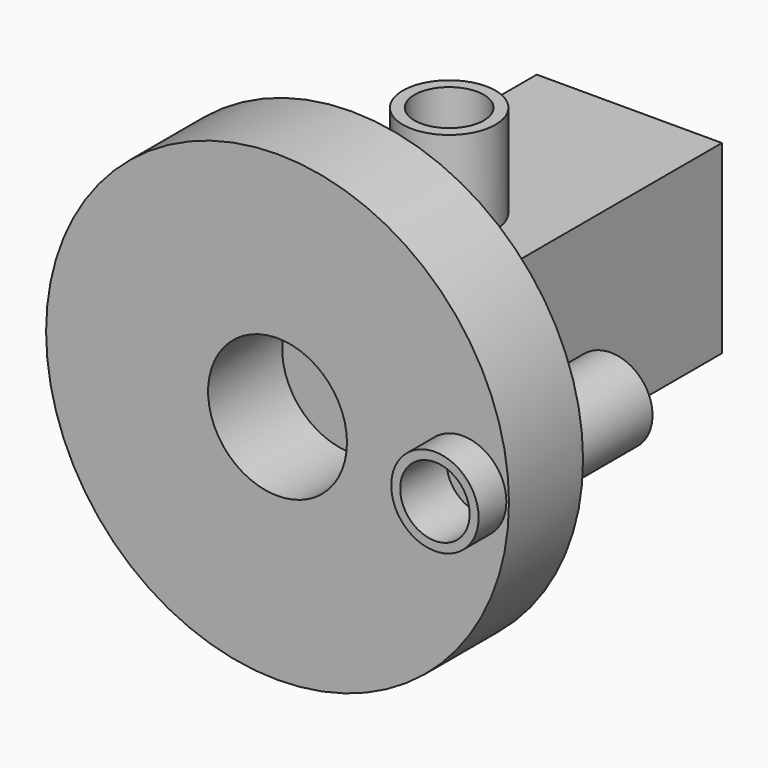
from build123d import *
from build123d import SkipClean  # not in build123d's __all__

# Parameters (mm, degrees)
F0_R      = 63.5
F1_DEPTH  = 25.4
F2_R      = 19.05
F3_DEPTH  = 25.401
F4_R      = 6.35
F5_DEPTH  = 25.4
F6_R      = 9.525
F7_DEPTH  = 6.35
F8_W      = 50.8
F8_H      = 50.8
F9_DEPTH  = 95.25
F10_R     = 19.05
F11_DEPTH = 88.9
F12_R     = 11.4435821265
F12_R_2   = 8.6754099319
F12_R_3   = 6.35
F13_DEPTH = 25.4
F14_R     = 12.7
F15_DEPTH = 25.4
F16_R     = 9.525
F17_DEPTH = 25.4
F18_R     = 11.9876896331
F18_R_2   = 9.525
F19_DEPTH = 9.525


# Not quite as in the source:
# - after a boolean that leaves OpenCascade's solid faulty, fix() repairs it


with BuildPart() as f1:
    # F0 (on Front) → F1 (new body)
    with BuildSketch(Plane.XZ):
        Circle(F0_R)
    extrude(amount=F1_DEPTH)

    # F2 (on face) → F3 (cut, through all)
    with BuildSketch(Plane.XZ.offset(25.4)):
        Circle(F2_R)
    extrude(amount=-F3_DEPTH, mode=Mode.SUBTRACT)

    # F4 (on face) → F5 (cut)
    with BuildSketch(Plane.XZ.offset(25.4)):
        with Locations((50.8, 0)):
            Circle(F4_R)
    extrude(amount=-F5_DEPTH, mode=Mode.SUBTRACT)

    # F6 (on face) → F7 (cut)
    with BuildSketch(Plane.XZ.offset(25.4)):
        with Locations((50.8, 0)):
            Circle(F6_R)
    extrude(amount=-F7_DEPTH, mode=Mode.SUBTRACT)

    # F8 (on face) → F9 (join)
    with BuildSketch(Plane(origin=(0, 0, 0), x_dir=(-1, 0, 0), z_dir=(0, 1, 0))):
        Rectangle(F8_W, F8_H)
    extrude(amount=F9_DEPTH)

    # F10 (on face) → F11 (cut)
    with BuildSketch(Plane(origin=(0, 95.25, 0), x_dir=(-1, 0, 0), z_dir=(0, 1, 0))):
        Circle(F10_R)
    extrude(amount=-F11_DEPTH, mode=Mode.SUBTRACT)

    # F12 (on face) → F13 (join)
    with BuildSketch(Plane(origin=(0, 0, 0), x_dir=(-1, 0, 0), z_dir=(0, 1, 0))):
        with Locations((-50.8, 0)):
            Circle(F12_R)
        with Locations((-50.8, 0)):
            Circle(F12_R_2, mode=Mode.SUBTRACT)
        with Locations((-50.8, 0)):
            Circle(F12_R_2)
        with Locations((-50.8, 0)):
            Circle(F12_R_3, mode=Mode.SUBTRACT)
    with SkipClean():  # cleaning this boolean's faces spoils the solid; the shape is the same uncleaned
        extrude(amount=F13_DEPTH)

    # F14 (on face) → F15 (join)
    with BuildSketch(Plane.XY.offset(25.4)):
        with Locations((0, 33.4604047239)):
            Circle(F14_R)
    extrude(amount=F15_DEPTH)

    add(f1.part.fix(), mode=Mode.REPLACE)

    # F16 (on face) → F17 (cut)
    with BuildSketch(Plane.XY.offset(50.8)):
        with Locations((0, 33.4604047239)):
            Circle(F16_R)
    extrude(amount=-F17_DEPTH, mode=Mode.SUBTRACT)

    add(f1.part.fix(), mode=Mode.REPLACE)

    # F18 (on face) → F19 (join)
    with BuildSketch(Plane.XZ.offset(25.4)):
        with Locations((50.8, 0)):
            Circle(F18_R)
        with Locations((50.8, 0)):
            Circle(F18_R_2, mode=Mode.SUBTRACT)
    extrude(amount=F19_DEPTH)


solid = f1.part
